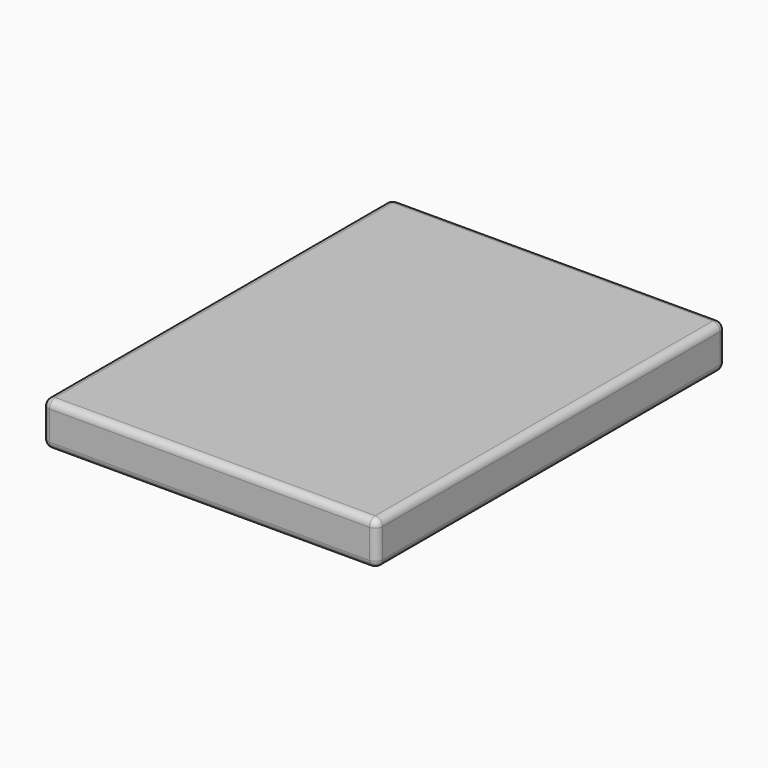
from build123d import *

# Parameters (mm, degrees)
F0_W     = 46
F0_H     = 6
F1_DEPTH = 60
F2_R     = 1


# Not quite as in the source:
# - a feature names something its author has since deleted; it is built from what else it names


with BuildPart() as f1:
    # F0 (on Front) → F1 (new body)
    with BuildSketch(Plane.XZ):
        with Locations((0, 3)):
            Rectangle(F0_W, F0_H)
    extrude(amount=-F1_DEPTH)

    # F2
    f2_edges = [f1.edges().sort_by_distance(p)[0] for p in [
        (0, 60, 6),
        (23, 30, 6),
        (-23, 30, 6),
        (0, 0, 6),
        (23, 60, 3),
        (-23, 60, 3),
        (0, 60, 0),
        (-23, 30, 0),
        (23, 30, 0),
        (0, 0, 0),
        (-23, 0, 3),
        (23, 0, 3),
    ]]
    fillet(f2_edges, radius=F2_R)


solid = f1.part
